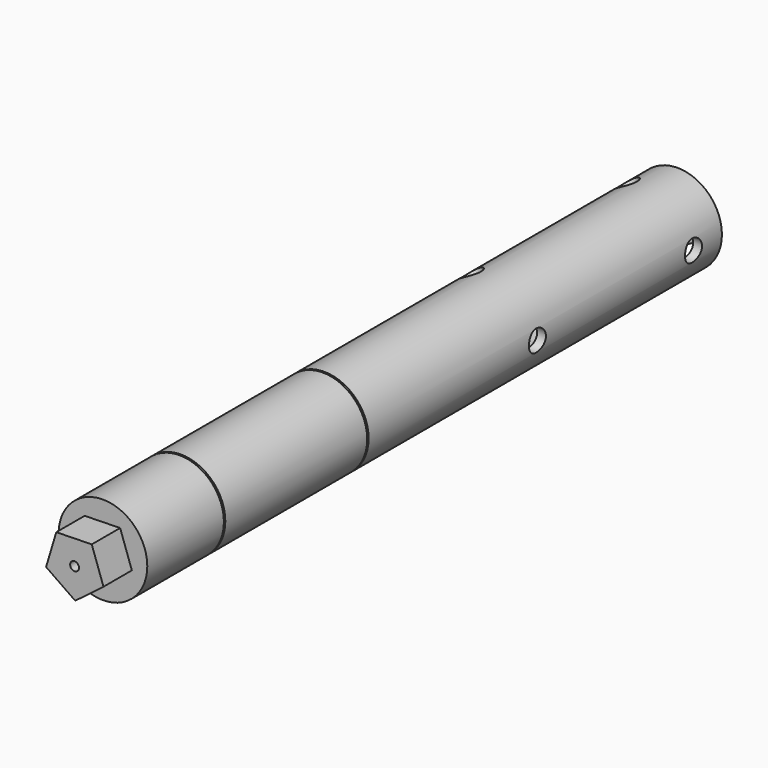
from build123d import *

# Parameters (mm, degrees)
F0_R          = 25
F0_R_2        = 20
F1_DEPTH      = 400
F2_R          = 25
F3_DEPTH      = 5
F5_DEPTH      = 20
F7_D          = 5
F10_D         = 12
F10_DEPTH     = 6
F10_START     = 0.7306779
F10_TIP       = 3.6051637142
F12_DEPTH     = 2
F17_D         = 12
F17_DEPTH     = 6
F17_START     = 0.7306779
F17_TIP       = 3.6051637142
F19_D         = 12
F19_DEPTH     = 6
F19_START     = 0.7306779
F19_TIP       = 3.6051637142
F21_R         = 25
F21_R_2       = 24
F22_DEPTH     = 1
F24_R         = 25
F24_R_2       = 24
F25_DEPTH     = 1
F27_DEPTH     = 20
F28_T1_DEPTH  = 16.0381401647
F28_T3_DEPTH  = 31.2249898061
F28_T5_DEPTH  = 16.0381402184
F28_T7_DEPTH  = 16.0381401647
F28_T9_DEPTH  = 31.2249898061
F28_T11_DEPTH = 16.0381402184
F28_T13_DEPTH = 16.0381401647
F28_T15_DEPTH = 31.2249898061
F28_T17_DEPTH = 16.0381402184


# Not quite as in the source:
# - a fillet or chamfer that OpenCascade refuses, or shapes differently, is made with other operations: its cross-section is extruded or revolved along the edge and cut away or added


with BuildPart() as f1:
    # F0 (on Front) → F1 (new body)
    with BuildSketch(Plane.XZ):
        Circle(F0_R)
        Circle(F0_R_2, mode=Mode.SUBTRACT)
    extrude(amount=F1_DEPTH)

    # F2 (on face) → F3 (join)
    with BuildSketch(Plane.XZ.offset(400)):
        Circle(F2_R)
    extrude(amount=F3_DEPTH)

    # F4 (on face) → F5 (join)
    with BuildSketch(Plane.XZ.offset(405)):
        Polygon((-16.0628025015, -5.6190539991), (0.380358971, -17.013016167), (16.2978772735, -4.8955682433), (9.6922831285, 13.9873885984), (-10.3077168715, 13.540249811), align=None)
    extrude(amount=F5_DEPTH)

    # F7 (through all)
    with Locations(Plane.XZ.offset(425)):
        with Locations((0, 0)):
            Hole(F7_D / 2)

    # F10
    # its depths count from where the whole tool has entered the part; down to there all is cleared
    with Locations(Plane.YZ.offset(25).offset(-F10_START)):
        with Locations((-20, 0), (-130, 0)):
            Hole(F10_D / 2, depth=F10_DEPTH)
            with Locations((0, 0, -(F10_DEPTH + F10_TIP / 2))):  # 118° drill point
                Cone(0, F10_D / 2, F10_TIP, mode=Mode.SUBTRACT)

    # F11 (on face) → F12 (join)
    with BuildSketch(Plane(origin=(0, 0, 0), x_dir=(-1, 0, 0), z_dir=(0, 1, 0))):
        Polygon((12.5, -21.6506350946), (12.5, 21.6506350946), (-25, 0), align=None)
    extrude(amount=F12_DEPTH)

    # F17
    # its depths count from where the whole tool has entered the part; down to there all is cleared
    with Locations(Plane(origin=(-12.5, 0, -21.6506350946), x_dir=(0.8660254038, 0, -0.5), z_dir=(-0.5, 0, -0.8660254038)).offset(-F17_START)):
        with Locations((0, 20), (0, 130)):
            Hole(F17_D / 2, depth=F17_DEPTH)
            with Locations((0, 0, -(F17_DEPTH + F17_TIP / 2))):  # 118° drill point
                Cone(0, F17_D / 2, F17_TIP, mode=Mode.SUBTRACT)

    # F19
    # its depths count from where the whole tool has entered the part; down to there all is cleared
    with Locations(Plane(origin=(-12.5, 0, 21.6506350946), x_dir=(0.8660254038, 0, 0.5), z_dir=(-0.5, 0, 0.8660254038)).offset(-F19_START)):
        with Locations((0, -20), (0, -130)):
            Hole(F19_D / 2, depth=F19_DEPTH)
            with Locations((0, 0, -(F19_DEPTH + F19_TIP / 2))):  # 118° drill point
                Cone(0, F19_D / 2, F19_TIP, mode=Mode.SUBTRACT)

    # F21 (on offset) → F22 (cut)
    with BuildSketch(Plane.XZ.offset(250)):
        Circle(F21_R)
        Circle(F21_R_2, mode=Mode.SUBTRACT)
    extrude(amount=-F22_DEPTH, mode=Mode.SUBTRACT)

    # F24 (on offset) → F25 (cut)
    with BuildSketch(Plane.XZ.offset(350)):
        Circle(F24_R)
        Circle(F24_R_2, mode=Mode.SUBTRACT)
    extrude(amount=F25_DEPTH, mode=Mode.SUBTRACT)

    # F26 (on face) → F27 (cut)
    with BuildSketch(Plane(origin=(0, 2, 0), x_dir=(-1, 0, 0), z_dir=(0, 1, 0))):
        Polygon((-20, 0), (10, -17.3205080757), (10, 17.3205080757), align=None)
    extrude(amount=-F27_DEPTH, mode=Mode.SUBTRACT)

    # F28: fillet of radius 5 on 3 edges, made by hand

    # F28_s2 → F28_t1 (cut)
    with BuildSketch(Plane(origin=(27.4102540378, 0, 15.8253175473), x_dir=(0, 1, 0), z_dir=(-0.8660254038, 0, -0.5))):
        with BuildLine():
            ThreePointArc((0, 12.5), (1.472135955, 10.7360679775), (2, 8.5))
            Line((2, 8.5), (2, 12.5))
            Line((2, 12.5), (0, 12.5))
        make_face()
    extrude(amount=F28_T1_DEPTH, mode=Mode.SUBTRACT)

    # F28_s4 → F28_t3 (cut)
    with BuildSketch(Plane(origin=(13.5208172258, 0, 7.806247465), x_dir=(0, 1, 0), z_dir=(-0.8660254038, 0, -0.5))):
        with BuildLine():
            ThreePointArc((0, 12.5), (1.472135955, 10.7360679775), (2, 8.5))
            Line((2, 8.5), (2, 12.5))
            Line((2, 12.5), (0, 12.5))
        make_face()
    extrude(amount=F28_T3_DEPTH, mode=Mode.SUBTRACT)

    # F28_s6 → F28_t5 (cut)
    with BuildSketch(Plane(origin=(-13.5208171792, 0, -7.8062474381), x_dir=(0, 1, 0), z_dir=(-0.8660254038, 0, -0.5))):
        with BuildLine():
            ThreePointArc((0, 12.5), (1.472135955, 10.7360679775), (2, 8.5))
            Line((2, 8.5), (2, 12.5))
            Line((2, 12.5), (0, 12.5))
        make_face()
    extrude(amount=F28_T5_DEPTH, mode=Mode.SUBTRACT)

    # F28_s8 → F28_t7 (cut)
    with BuildSketch(Plane.XY.offset(-31.6506350946)):
        with BuildLine():
            ThreePointArc((-12.5, 0), (-10.7360679775, 1.472135955), (-8.5, 2))
            Line((-8.5, 2), (-12.5, 2))
            Line((-12.5, 2), (-12.5, 0))
        make_face()
    extrude(amount=F28_T7_DEPTH, mode=Mode.SUBTRACT)

    # F28_s10 → F28_t9 (cut)
    with BuildSketch(Plane.XY.offset(-15.61249493)):
        with BuildLine():
            ThreePointArc((-12.5, 0), (-10.7360679775, 1.472135955), (-8.5, 2))
            Line((-8.5, 2), (-12.5, 2))
            Line((-12.5, 2), (-12.5, 0))
        make_face()
    extrude(amount=F28_T9_DEPTH, mode=Mode.SUBTRACT)

    # F28_s12 → F28_t11 (cut)
    with BuildSketch(Plane.XY.offset(15.6124948762)):
        with BuildLine():
            ThreePointArc((-12.5, 0), (-10.7360679775, 1.472135955), (-8.5, 2))
            Line((-8.5, 2), (-12.5, 2))
            Line((-12.5, 2), (-12.5, 0))
        make_face()
    extrude(amount=F28_T11_DEPTH, mode=Mode.SUBTRACT)

    # F28_s14 → F28_t13 (cut)
    with BuildSketch(Plane(origin=(-27.4102540378, 0, 15.8253175473), x_dir=(0, 1, 0), z_dir=(0.8660254038, 0, -0.5))):
        with BuildLine():
            ThreePointArc((0, 12.5), (1.472135955, 10.7360679775), (2, 8.5))
            Line((2, 8.5), (2, 12.5))
            Line((2, 12.5), (0, 12.5))
        make_face()
    extrude(amount=F28_T13_DEPTH, mode=Mode.SUBTRACT)

    # F28_s16 → F28_t15 (cut)
    with BuildSketch(Plane(origin=(-13.5208172258, 0, 7.806247465), x_dir=(0, 1, 0), z_dir=(0.8660254038, 0, -0.5))):
        with BuildLine():
            ThreePointArc((0, 12.5), (1.472135955, 10.7360679775), (2, 8.5))
            Line((2, 8.5), (2, 12.5))
            Line((2, 12.5), (0, 12.5))
        make_face()
    extrude(amount=F28_T15_DEPTH, mode=Mode.SUBTRACT)

    # F28_s18 → F28_t17 (cut)
    with BuildSketch(Plane(origin=(13.5208171792, 0, -7.8062474381), x_dir=(0, 1, 0), z_dir=(0.8660254038, 0, -0.5))):
        with BuildLine():
            ThreePointArc((0, 12.5), (1.472135955, 10.7360679775), (2, 8.5))
            Line((2, 8.5), (2, 12.5))
            Line((2, 12.5), (0, 12.5))
        make_face()
    extrude(amount=F28_T17_DEPTH, mode=Mode.SUBTRACT)


solid = f1.part
